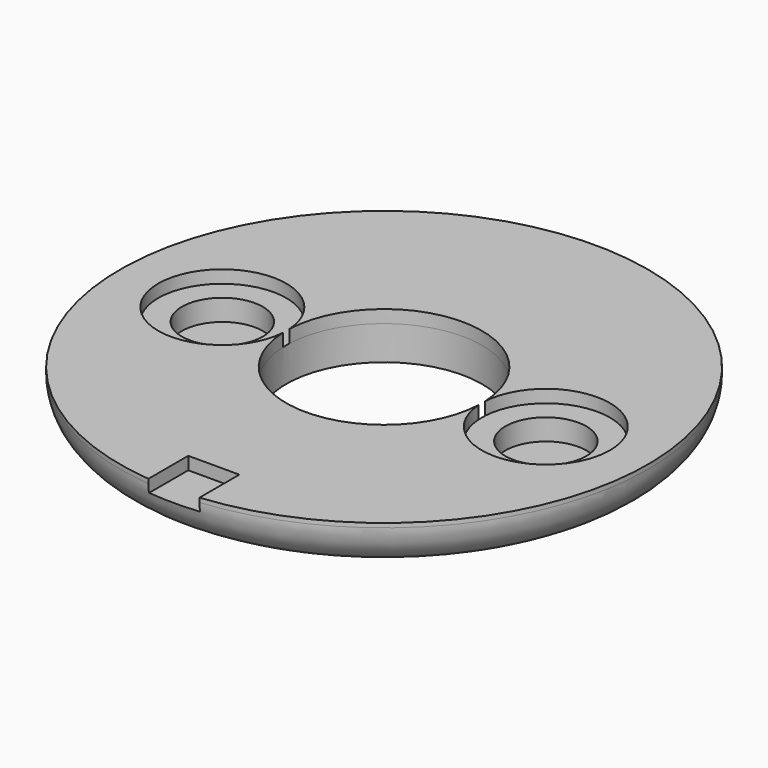
from build123d import *
from build123d import SkipClean  # not in build123d's __all__

# Parameters (mm, degrees)
F0_R     = 31
F0_R_2   = 11.5
F1_DEPTH = 1.5
F2_R     = 31
F2_R_2   = 4.75
F2_R_3   = 11.5
F3_DEPTH = 4
F5_DEPTH = 1.5


# Not quite as in the source:
# - a fillet or chamfer that OpenCascade refuses, or shapes differently, is made with other operations: its cross-section is extruded or revolved along the edge and cut away or added


with BuildPart() as f1:
    # F0 (on Top) → F1 (new body)
    with BuildSketch(Plane.XY):
        Circle(F0_R)
        Circle(F0_R_2, mode=Mode.SUBTRACT)
    extrude(amount=-F1_DEPTH)

    # F2 (on face) → F3 (join)
    with BuildSketch(Plane(origin=(0, 0, -1.5), x_dir=(1, 0, 0), z_dir=(0, 0, -1))):
        Circle(F2_R)
        with Locations((-19, 0)):
            Circle(F2_R_2, mode=Mode.SUBTRACT)
        Circle(F2_R_3, mode=Mode.SUBTRACT)
        with Locations((19, 0)):
            Circle(F2_R_2, mode=Mode.SUBTRACT)
    extrude(amount=-F3_DEPTH)

    # F4 (on face) → F5 (join)
    with BuildSketch(Plane.XY.offset(2.5)):
        with BuildLine():
            ThreePointArc((3, -30.8544972411), (22.9564805665, -20.832666656), (31, 0))
            ThreePointArc((31, 0), (-20.832666656, 22.9564805665), (-3, -30.8544972411))
            Line((-3, -30.8544972411), (-3, -25))
            Line((-3, -25), (3, -25))
            Line((3, -25), (3, -30.8544972411))
        make_face()
        with BuildLine():
            ThreePointArc((-11.4901151316, 0.4767119288), (0, 11.5), (11.4901151316, 0.4767119288))
            ThreePointArc((11.4901151316, 0.4767119288), (19.2384757484, 7.5212202678), (26.525, 0))
            ThreePointArc((26.525, 0), (19.2384757484, -7.5212202678), (11.4901151316, -0.4767119288))
            ThreePointArc((11.4901151316, -0.4767119288), (0, -11.5), (-11.4901151316, -0.4767119288))
            ThreePointArc((-11.4901151316, -0.4767119288), (-26.525, 0), (-11.4901151316, 0.4767119288))
        make_face(mode=Mode.SUBTRACT)
    with SkipClean():  # cleaning this boolean's faces spoils the solid; the shape is the same uncleaned
        extrude(amount=F5_DEPTH)

    # F6: fillet of radius 5 on 1 edges, made by hand

    # F6_s1 → F6_t2 (revolve, cut)
    with BuildSketch(Plane.XZ):
        with BuildLine():
            ThreePointArc((31, 3.5), (29.5355339059, -0.0355339059), (26, -1.5))
            Line((26, -1.5), (31, -1.5))
            Line((31, -1.5), (31, 3.5))
        make_face()
    revolve(axis=Axis((0, 0, -1.5), (0, 0, 1)), mode=Mode.SUBTRACT)


solid = f1.part
